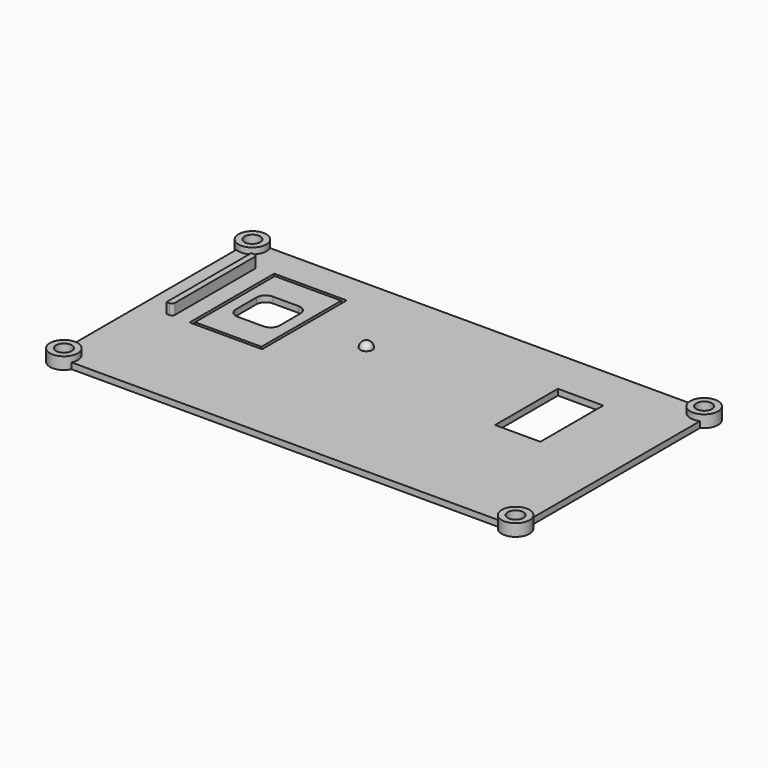
from build123d import *

# Parameters (mm, degrees)
F0_W           = 153.5
F0_H           = 82
F1_DEPTH       = 2
F2_W           = 15
F2_H           = 26
F2_W_2         = 14.5
F2_H_2         = 14.5
F3_DEPTH       = 2.001
F4_R           = 2
F5_DEPTH       = 2
F6_R           = 1.99999
F7_W           = 24
F7_H           = 35
F7_W_2         = 22
F7_H_2         = 33
F8_DEPTH       = 1
F10_R          = 4.6
F10_R_2        = 2.6
F11_DEPTH      = 4
F12_R          = 2.6
F13_DEPTH      = 4.001
F14_W          = 2
F14_H          = 35
F15_DEPTH      = 2
F15_DEPTH_BACK = 1.5
F16_R          = 1
F17_R          = 3


# Not quite as in the source:
# - a fillet or chamfer is up to 0.001 mm smaller than in the source, because OpenCascade refuses the exact size
# - a feature names something its author has since deleted; it is built from what else it names


with BuildPart() as f1:
    # F0 (on Top) → F1 (new body)
    with BuildSketch(Plane.XY):
        Rectangle(F0_W, F0_H)
    extrude(amount=F1_DEPTH)

    # F2 (on face) → F3 (cut, through all)
    with BuildSketch(Plane.XY.offset(2)):
        with Locations((44.25, 13)):
            Rectangle(F2_W, F2_H)
        with Locations((-48.75, 13)):
            Rectangle(F2_W_2, F2_H_2)
    extrude(amount=-F3_DEPTH, mode=Mode.SUBTRACT)

    # F4 (on face) → F5 (join)
    with BuildSketch(Plane.XY.offset(2)):
        with Locations((-16.25, 13)):
            Circle(F4_R)
    extrude(amount=F5_DEPTH)

    # F6 (radius 2 in the source; OpenCascade refuses exactly that, so slightly less here)
    f6_edges = [f1.edges().sort_by_distance(p)[0] for p in [
        (-18.25, 13, 4),
    ]]
    fillet(f6_edges, radius=F6_R)

    # F7 (on face) → F8 (cut)
    with BuildSketch(Plane.XY.offset(2)):
        with Locations((-48.75, 13)):
            Rectangle(F7_W, F7_H)
        with Locations((-48.75, 13)):
            Rectangle(F7_W_2, F7_H_2, mode=Mode.SUBTRACT)
    extrude(amount=-F8_DEPTH, mode=Mode.SUBTRACT)

    # F10 (on offset) → F11 (join)
    with BuildSketch(Plane.XY.offset(4)):
        with Locations((-74.75, 39)):
            Circle(F10_R)
        with Locations((-74.75, 39)):
            Circle(F10_R_2, mode=Mode.SUBTRACT)
        with Locations((74.75, 39)):
            Circle(F10_R)
        with Locations((74.75, 39)):
            Circle(F10_R_2, mode=Mode.SUBTRACT)
        with Locations((-74.75, -39)):
            Circle(F10_R)
        with Locations((-74.75, -39)):
            Circle(F10_R_2, mode=Mode.SUBTRACT)
        with Locations((74.75, -39)):
            Circle(F10_R)
        with Locations((74.75, -39)):
            Circle(F10_R_2, mode=Mode.SUBTRACT)
    extrude(amount=-F11_DEPTH)

    # F12 (on face) → F13 (cut, through all)
    with BuildSketch(Plane.XY.offset(4)):
        with Locations((-74.75, 39)):
            Circle(F12_R)
        with Locations((74.75, 39)):
            Circle(F12_R)
        with Locations((-74.75, -39)):
            Circle(F12_R)
        with Locations((74.75, -39)):
            Circle(F12_R)
    extrude(amount=-F13_DEPTH, mode=Mode.SUBTRACT)

    # F14 (on offset) → F15 (join, two sides)
    with BuildSketch(Plane.XY.offset(4)) as f15_sk:
        with Locations((-67.35, 13)):
            Rectangle(F14_W, F14_H)
    extrude(amount=-F15_DEPTH)
    extrude(f15_sk.sketch, amount=F15_DEPTH_BACK)

    # F16
    f16_edges = [f1.edges().sort_by_distance(p)[0] for p in [
        (-66.35, -4.5, 3.75),
        (-66.35, 30.5, 3.75),
    ]]
    fillet(f16_edges, radius=F16_R)

    # F17
    f17_edges = [f1.edges().sort_by_distance(p)[0] for p in [
        (-56, 20.25, 1),
        (-41.5, 5.75, 1),
        (-56, 5.75, 1),
        (-41.5, 20.25, 1),
    ]]
    fillet(f17_edges, radius=F17_R)


solid = f1.part
